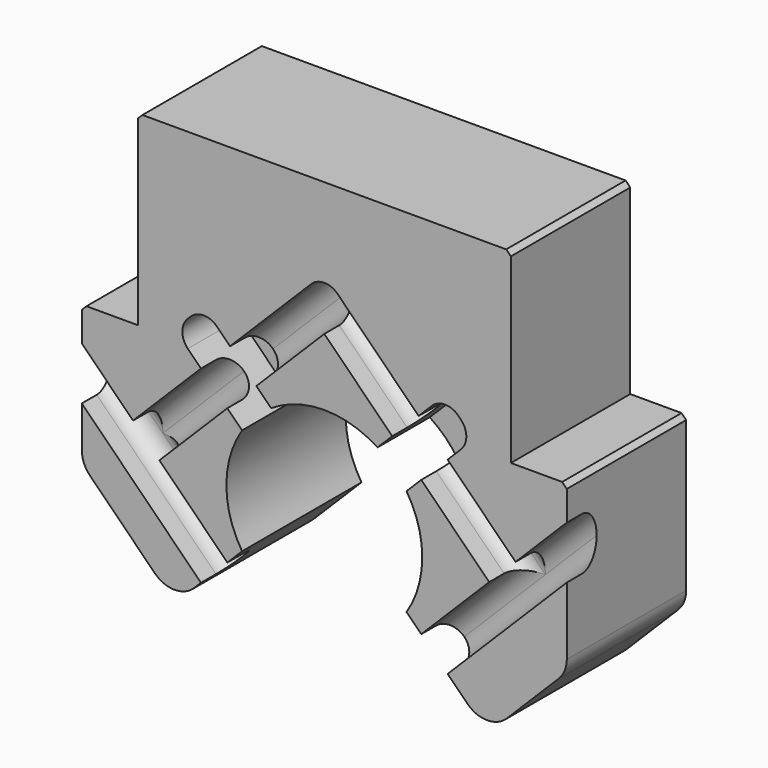
from build123d import *

# Parameters (mm, degrees)
F1_DEPTH = 16
F2_DEPTH = 7
F3_DEPTH = 4
F4_R     = 2
F5_R     = 1.9999
F6_R     = 3
F7_SIZE  = 0.5


# Not quite as in the source:
# - a fillet or chamfer is up to 0.001 mm smaller than in the source, because OpenCascade refuses the exact size
# - a feature names something its author has since deleted; it is built from what else it names


with BuildPart() as f1:
    # F0 (on Front) → F1 (new body)
    with BuildSketch(Plane.XZ):
        with BuildLine():
            ThreePointArc((-5.7041860158, 8.815455853), (0, 10.5), (5.7041860158, 8.815455853))
            Line((5.7041860158, 8.815455853), (7.2831998462, 10.3944696834))
            Line((7.2831998462, 10.3944696834), (0, 17.6776695297))
            Line((0, 17.6776695297), (-7.2831998462, 10.3944696834))
            Line((-7.2831998462, 10.3944696834), (-5.7041860158, 8.815455853))
        make_face()
        with BuildLine():
            ThreePointArc((-8.815455853, 5.7041860158), (-7.4246212025, 7.4246212025), (-5.7041860158, 8.815455853))
            Line((-5.7041860158, 8.815455853), (-7.2831998462, 10.3944696834))
            Line((-7.2831998462, 10.3944696834), (-10.3944696834, 7.2831998462))
            Line((-10.3944696834, 7.2831998462), (-8.815455853, 5.7041860158))
        make_face()
        with BuildLine():
            ThreePointArc((-8.815455853, -5.7041860158), (-10.5, 0), (-8.815455853, 5.7041860158))
            Line((-8.815455853, 5.7041860158), (-10.3944696834, 7.2831998462))
            Line((-10.3944696834, 7.2831998462), (-17.6776695297, 0))
            Line((-17.6776695297, 0), (-10.3944696834, -7.2831998462))
            Line((-10.3944696834, -7.2831998462), (-8.815455853, -5.7041860158))
        make_face()
        with BuildLine():
            ThreePointArc((5.7041860158, 8.815455853), (7.4246212025, 7.4246212025), (8.815455853, 5.7041860158))
            Line((8.815455853, 5.7041860158), (10.3944696834, 7.2831998462))
            Line((10.3944696834, 7.2831998462), (7.2831998462, 10.3944696834))
            Line((7.2831998462, 10.3944696834), (5.7041860158, 8.815455853))
        make_face()
        Polygon((0, 17.6776695297), (7.2831998462, 10.3944696834), (10.111626971, 13.2228968082), (0, 23.3345237792), (-10.111626971, 13.2228968082), (-7.2831998462, 10.3944696834), align=None)
        Polygon((7.2831998462, 10.3944696834), (10.3944696834, 7.2831998462), (13.2228968082, 10.111626971), (10.111626971, 13.2228968082), align=None)
        Polygon((-10.3944696834, 7.2831998462), (-7.2831998462, 10.3944696834), (-10.111626971, 13.2228968082), (-13.2228968082, 10.111626971), align=None)
        Polygon((-17.6776695297, 0), (-10.3944696834, 7.2831998462), (-13.2228968082, 10.111626971), (-20.5060966544, 2.8284271247), (-26, 8.3223304703), (-26, 2.6654762208), (-13.2228968082, -10.111626971), (-10.3944696834, -7.2831998462), align=None)
        Polygon((-13.2228968082, 10.111626971), (-10.111626971, 13.2228968082), (-12.9400540957, 16.0513239329), (-16.0513239329, 12.9400540957), align=None)
        Polygon((17.6776695297, 0), (10.3944696834, -7.2831998462), (13.2228968082, -10.111626971), (26, 2.6654762208), (26, 8.3223304703), (20.5060966544, 2.8284271247), (13.2228968082, 10.111626971), (10.3944696834, 7.2831998462), align=None)
        with BuildLine():
            ThreePointArc((8.815455853, 5.7041860158), (10.5, 0), (8.815455853, -5.7041860158))
            Line((8.815455853, -5.7041860158), (10.3944696834, -7.2831998462))
            Line((10.3944696834, -7.2831998462), (17.6776695297, 0))
            Line((17.6776695297, 0), (10.3944696834, 7.2831998462))
            Line((10.3944696834, 7.2831998462), (8.815455853, 5.7041860158))
        make_face()
        Polygon((16.0513239329, 12.9400540957), (13.2228968082, 10.111626971), (20.5060966544, 2.8284271247), (26, 8.3223304703), (26, 12), (20, 12), (20, 32), (0, 32), (-20, 32), (-20, 12), (-26, 12), (-26, 8.3223304703), (-20.5060966544, 2.8284271247), (-13.2228968082, 10.111626971), (-16.0513239329, 12.9400540957), (-12.9400540957, 16.0513239329), (-10.111626971, 13.2228968082), (0, 23.3345237792), (10.111626971, 13.2228968082), (12.9400540957, 16.0513239329), align=None)
        Polygon((10.111626971, 13.2228968082), (13.2228968082, 10.111626971), (16.0513239329, 12.9400540957), (12.9400540957, 16.0513239329), align=None)
        Polygon((26, 2.6654762208), (13.2228968082, -10.111626971), (17.4655374953, -14.3542676581), (26, -5.8198051534), align=None)
        Polygon((-16.0513239329, -12.9400540957), (-13.2228968082, -10.111626971), (-26, 2.6654762208), (-26, -2.9913780286), align=None)
    extrude(amount=-F1_DEPTH)

    # F0 (on Front) → F2 (cut)
    with BuildSketch(Plane.XZ):
        Polygon((10.111626971, 13.2228968082), (13.2228968082, 10.111626971), (16.0513239329, 12.9400540957), (12.9400540957, 16.0513239329), align=None)
        Polygon((7.2831998462, 10.3944696834), (10.3944696834, 7.2831998462), (13.2228968082, 10.111626971), (10.111626971, 13.2228968082), align=None)
        with BuildLine():
            ThreePointArc((5.7041860158, 8.815455853), (7.4246212025, 7.4246212025), (8.815455853, 5.7041860158))
            Line((8.815455853, 5.7041860158), (10.3944696834, 7.2831998462))
            Line((10.3944696834, 7.2831998462), (7.2831998462, 10.3944696834))
            Line((7.2831998462, 10.3944696834), (5.7041860158, 8.815455853))
        make_face()
        with BuildLine():
            ThreePointArc((-8.815455853, 5.7041860158), (-7.4246212025, 7.4246212025), (-5.7041860158, 8.815455853))
            Line((-5.7041860158, 8.815455853), (-7.2831998462, 10.3944696834))
            Line((-7.2831998462, 10.3944696834), (-10.3944696834, 7.2831998462))
            Line((-10.3944696834, 7.2831998462), (-8.815455853, 5.7041860158))
        make_face()
        Polygon((-13.2228968082, 10.111626971), (-10.111626971, 13.2228968082), (-12.9400540957, 16.0513239329), (-16.0513239329, 12.9400540957), align=None)
        Polygon((-10.3944696834, 7.2831998462), (-7.2831998462, 10.3944696834), (-10.111626971, 13.2228968082), (-13.2228968082, 10.111626971), align=None)
    extrude(amount=-F2_DEPTH, mode=Mode.SUBTRACT)

    # F0 (on Front) → F3 (cut)
    with BuildSketch(Plane.XZ):
        Polygon((0, 17.6776695297), (7.2831998462, 10.3944696834), (10.111626971, 13.2228968082), (0, 23.3345237792), (-10.111626971, 13.2228968082), (-7.2831998462, 10.3944696834), align=None)
        Polygon((17.6776695297, 0), (10.3944696834, -7.2831998462), (13.2228968082, -10.111626971), (26, 2.6654762208), (26, 8.3223304703), (20.5060966544, 2.8284271247), (13.2228968082, 10.111626971), (10.3944696834, 7.2831998462), align=None)
        Polygon((-17.6776695297, 0), (-10.3944696834, 7.2831998462), (-13.2228968082, 10.111626971), (-20.5060966544, 2.8284271247), (-26, 8.3223304703), (-26, 2.6654762208), (-13.2228968082, -10.111626971), (-10.3944696834, -7.2831998462), align=None)
    extrude(amount=-F3_DEPTH, mode=Mode.SUBTRACT)

    # F4
    f4_edges = [f1.edges().sort_by_distance(p)[0] for p in [
        (-16.051324, 3.5, 12.940054),
        (-12.940054, 3.5, 16.051324),
        (12.940054, 3.5, 16.051324),
        (16.051324, 3.5, 12.940054),
        (0, 2, 23.334524),
    ]]
    fillet(f4_edges, radius=F4_R)

    # F5 (radius 2 in the source; OpenCascade refuses exactly that, so slightly less here)
    f5_edges = [f1.edges().sort_by_distance(p)[0] for p in [
        (19.611448, 4, -3.723075),
        (14.03607, 4, -3.6416),
        (14.03607, 4, 3.6416),
        (16.864497, 4, 6.470027),
        (5.76292, 4, 17.571604),
        (-16.864497, 4, 6.470027),
        (-23.253048, 4, 5.575379),
        (-14.03607, 4, -3.6416),
        (-3.6416, 4, 14.03607),
        (-14.03607, 4, 3.6416),
        (-19.611448, 4, -3.723075),
        (23.253048, 4, 5.575379),
        (0, 4, 22.506097),
        (-5.76292, 4, 17.571604),
        (3.6416, 4, 14.03607),
    ]]
    fillet(f5_edges, radius=F5_R)

    # F6
    f6_edges = [f1.edges().sort_by_distance(p)[0] for p in [
        (17.465537, 8, -14.354268),
        (-16.051324, 8, -12.940054),
        (26, 8, -5.819805),
        (-26, 8, -2.991378),
    ]]
    fillet(f6_edges, radius=F6_R)

    # F7
    f7_edges = [f1.edges().sort_by_distance(p)[0] for p in [
        (20, 8, 32),
        (26, 8, 12),
        (-20, 8, 32),
        (-26, 8, 12),
    ]]
    chamfer(f7_edges, length=F7_SIZE)


solid = f1.part
